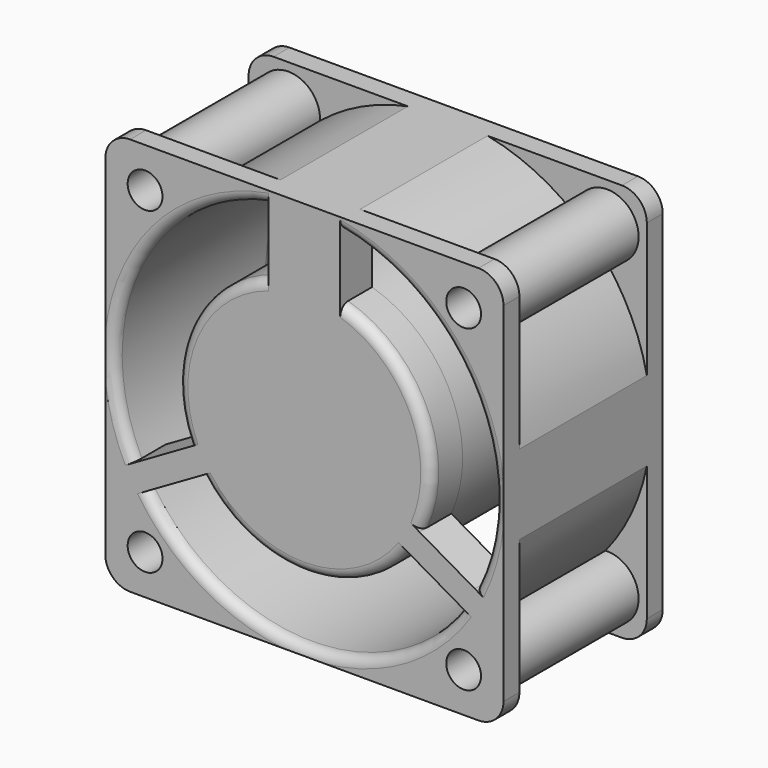
from build123d import *

# Parameters (mm, degrees)
F0_W         = 40
F0_H         = 40
F0_R         = 1.75
F0_R_2       = 19.1
F1_DEPTH     = 10
F3_DEPTH     = 8
F4_R         = 2.5
F6_DEPTH     = 4
F7_W         = 18
F7_H         = 12.7
F9_T6_ANGLE  = 120.5658801398
F9_T11_ANGLE = 120.5658801398
F9_T17_ANGLE = 120.5658801398
F9_T23_ANGLE = 120.5658801398
F9_T28_ANGLE = 131.5003349081
F9_T33_ANGLE = 131.5003349081
F9_T39_ANGLE = 131.5003349081
F9_T44_ANGLE = 120.4657257073
F9_T50_ANGLE = 120.4657257073
F9_T55_ANGLE = 86.6375868427
F9_T60_ANGLE = 127.6538287978
F9_T65_ANGLE = 127.6538287978
F9_T71_ANGLE = 127.6538287978
F9_T78_ANGLE = 33.8224519286
F9_T83_ANGLE = 33.8224519286


# Not quite as in the source:
# - a fillet or chamfer that OpenCascade refuses, or shapes differently, is made with other operations: its cross-section is extruded or revolved along the edge and cut away or added


with BuildPart() as f1:
    # F0 (on Front) → F1 (new body, symmetric)
    with BuildSketch(Plane.XZ):
        Rectangle(F0_W, F0_H)
        with Locations((-16, -16)):
            Circle(F0_R, mode=Mode.SUBTRACT)
        with Locations((16, -16)):
            Circle(F0_R, mode=Mode.SUBTRACT)
        with Locations((-16, 16)):
            Circle(F0_R, mode=Mode.SUBTRACT)
        Circle(F0_R_2, mode=Mode.SUBTRACT)
        with Locations((16, 16)):
            Circle(F0_R, mode=Mode.SUBTRACT)
    extrude(amount=F1_DEPTH, both=True)

    # F2 (on Front) → F3 (cut, symmetric)
    with BuildSketch(Plane.XZ):
        with BuildLine():
            ThreePointArc((-15.8567471072, 12.8282333616), (-18.2450640303, 18.2450640303), (-12.8282333616, 15.8567471072))
            ThreePointArc((-12.8282333616, 15.8567471072), (-8.6653906808, 18.463775463), (-4, 20))
            Line((-4, 20), (-4, 20.3960780544))
            Line((-4, 20.3960780544), (-20.3960780544, 20.3960780544))
            Line((-20.3960780544, 20.3960780544), (-20.3960780544, 4))
            Line((-20.3960780544, 4), (-20, 4))
            ThreePointArc((-20, 4), (-18.463775463, 8.6653906808), (-15.8567471072, 12.8282333616))
        make_face()
        with BuildLine():
            Line((20.3960780544, 4), (20.3960780544, 20.3960780544))
            Line((20.3960780544, 20.3960780544), (4, 20.3960780544))
            Line((4, 20.3960780544), (4, 20))
            ThreePointArc((4, 20), (8.6653906808, 18.463775463), (12.8282333616, 15.8567471072))
            ThreePointArc((12.8282333616, 15.8567471072), (18.2450640303, 18.2450640303), (15.8567471072, 12.8282333616))
            ThreePointArc((15.8567471072, 12.8282333616), (18.463775463, 8.6653906808), (20, 4))
            Line((20, 4), (20.3960780544, 4))
        make_face()
        with BuildLine():
            Line((-20.3960780544, -4), (-20.3960780544, -20.3960780544))
            Line((-20.3960780544, -20.3960780544), (-4, -20.3960780544))
            Line((-4, -20.3960780544), (-4, -20))
            ThreePointArc((-4, -20), (-8.6653906808, -18.463775463), (-12.8282333616, -15.8567471072))
            ThreePointArc((-12.8282333616, -15.8567471072), (-18.2450640303, -18.2450640303), (-15.8567471072, -12.8282333616))
            ThreePointArc((-15.8567471072, -12.8282333616), (-18.463775463, -8.6653906808), (-20, -4))
            Line((-20, -4), (-20.3960780544, -4))
        make_face()
        with BuildLine():
            Line((4, -20.3960780544), (20.3960780544, -20.3960780544))
            Line((20.3960780544, -20.3960780544), (20.3960780544, -4))
            Line((20.3960780544, -4), (20, -4))
            ThreePointArc((20, -4), (18.463775463, -8.6653906808), (15.8567471072, -12.8282333616))
            ThreePointArc((15.8567471072, -12.8282333616), (18.2450640303, -18.2450640303), (12.8282333616, -15.8567471072))
            ThreePointArc((12.8282333616, -15.8567471072), (8.6653906808, -18.463775463), (4, -20))
            Line((4, -20), (4, -20.3960780544))
        make_face()
    extrude(amount=F3_DEPTH, both=True, mode=Mode.SUBTRACT)

    # F4
    f4_edges = [f1.edges().sort_by_distance(p)[0] for p in [
        (20, -9, 20),
        (20, 9, 20),
        (20, -9, -20),
        (20, 9, -20),
        (-20, -9, 20),
        (-20, 9, 20),
        (-20, 9, -20),
        (-20, -9, -20),
    ]]
    fillet(f4_edges, radius=F4_R)

    # F5 (on face) → F6 (join)
    with BuildSketch(Plane.XZ.offset(10)):
        with BuildLine():
            Line((-3.6, 18.7576650999), (-3.6, 12.1790804251))
            ThreePointArc((-3.6, 12.1790804251), (-11.5533772944, 5.2734687913), (-11.5597385217, -5.2595099877))
            Line((-11.5597385217, -5.2595099877), (-17.1195297525, -8.4694569515))
            ThreePointArc((-17.1195297525, -8.4694569515), (-16.5410852123, -9.55), (-15.8945297525, -10.5912191908))
            Line((-15.8945297525, -10.5912191908), (-10.3347385217, -7.381272227))
            ThreePointArc((-10.3347385217, -7.381272227), (0, -12.7), (10.3347385217, -7.381272227))
            Line((10.3347385217, -7.381272227), (15.8945297525, -10.5912191908))
            ThreePointArc((15.8945297525, -10.5912191908), (16.5410852123, -9.55), (17.1195297525, -8.4694569515))
            Line((17.1195297525, -8.4694569515), (11.5597385217, -5.2595099877))
            ThreePointArc((11.5597385217, -5.2595099877), (11.5533772944, 5.2734687913), (3.6, 12.1790804251))
            Line((3.6, 12.1790804251), (3.6, 18.7576650999))
            ThreePointArc((3.6, 18.7576650999), (0, 19.1), (-3.6, 18.7576650999))
        make_face()
    extrude(amount=-F6_DEPTH)

    # F7 (on Right) → F8 (revolve)
    with BuildSketch(Plane.YZ):
        with Locations((1, 6.35)):
            Rectangle(F7_W, F7_H)
    revolve(axis=Axis((0, 1.2222109362, 0), (0, 1, 0)))

    # F9: fillet of radius 1 on 9 edges, made by hand

    # F9_s1 → F9_t2 (revolve, cut)
    with BuildSketch(Plane.YZ):
        with BuildLine():
            ThreePointArc((9, 12.7), (9.7071067812, 12.4071067812), (10, 11.7))
            Line((10, 11.7), (10, 12.7))
            Line((10, 12.7), (9, 12.7))
        make_face()
    revolve(axis=Axis((0, 10, 0), (0, 1, 0)), mode=Mode.SUBTRACT)


with BuildPart() as f9_tool4:
    # F9_s5 → F9_t6 (revolve)
    with BuildSketch(Plane(origin=(0, 0, 0), x_dir=(0, 1, 0), z_dir=(-0.5842341064, 0, -0.8115851828))):
        with BuildLine():
            ThreePointArc((-10, 11.7), (-9.7071067812, 12.4071067812), (-9, 12.7))
            Line((-9, 12.7), (-10, 12.7))
            Line((-10, 12.7), (-10, 11.7))
        make_face()
    revolve(axis=Axis((0, -10, 0), (0, -1, 0)), revolution_arc=F9_T6_ANGLE)

    split(bisect_by=Plane(origin=(-0.6125, 0, -1.0608811196), x_dir=(0, 1, 0), z_dir=(-0.5, 0, -0.8660254038)), keep=Keep.TOP)


with BuildPart() as f1_1:
    add(f1.part)

    # F9_t3: cut F9_tool4
    add(f9_tool4.part, mode=Mode.SUBTRACT)


with BuildPart() as f9_tool9:
    # F9_s10 → F9_t11 (revolve)
    with BuildSketch(Plane(origin=(0, 0, 0), x_dir=(0, 1, 0), z_dir=(-0.5842341064, 0, -0.8115851828))):
        with BuildLine():
            ThreePointArc((-10, 11.7), (-9.7071067812, 12.4071067812), (-9, 12.7))
            Line((-9, 12.7), (-10, 12.7))
            Line((-10, 12.7), (-10, 11.7))
        make_face()
    revolve(axis=Axis((0, -10, 0), (0, -1, 0)), revolution_arc=F9_T11_ANGLE)

    split(bisect_by=Plane.YZ.offset(3.6), keep=Keep.TOP)

    split(bisect_by=Plane(origin=(0.6125, 0, 1.0608811196), x_dir=(0, 1, 0), z_dir=(0.5, 0, 0.8660254038)), keep=Keep.TOP)


with BuildPart() as f1_2:
    add(f1_1.part)

    # F9_t8: cut F9_tool9
    add(f9_tool9.part, mode=Mode.SUBTRACT)


with BuildPart() as f9_tool15:
    # F9_s16 → F9_t17 (revolve)
    with BuildSketch(Plane(origin=(0, 0, 0), x_dir=(0, 1, 0), z_dir=(0.9959112122, 0, 0.0903374635))):
        with BuildLine():
            ThreePointArc((-10, 11.7), (-9.7071067812, 12.4071067812), (-9, 12.7))
            Line((-9, 12.7), (-10, 12.7))
            Line((-10, 12.7), (-10, 11.7))
        make_face()
    revolve(axis=Axis((0, -10, 0), (0, -1, 0)), revolution_arc=F9_T17_ANGLE)

    split(bisect_by=Plane(origin=(-0.6125, 0, 1.0608811196), x_dir=(0, 1, 0), z_dir=(-0.5, 0, 0.8660254038)), keep=Keep.TOP)

    split(bisect_by=Plane.YZ.offset(-3.6), keep=Keep.BOTTOM)


with BuildPart() as f1_3:
    add(f1_2.part)

    # F9_t14: cut F9_tool15
    add(f9_tool15.part, mode=Mode.SUBTRACT)


with BuildPart() as f9_tool21:
    # F9_s22 → F9_t23 (revolve)
    with BuildSketch(Plane(origin=(0, 0, 0), x_dir=(0, 1, 0), z_dir=(0.9959112122, 0, 0.0903374635))):
        with BuildLine():
            ThreePointArc((-10, 11.7), (-9.7071067812, 12.4071067812), (-9, 12.7))
            Line((-9, 12.7), (-10, 12.7))
            Line((-10, 12.7), (-10, 11.7))
        make_face()
    revolve(axis=Axis((0, -10, 0), (0, -1, 0)), revolution_arc=F9_T23_ANGLE)

    split(bisect_by=Plane(origin=(0.6125, 0, -1.0608811196), x_dir=(0, 1, 0), z_dir=(0.5, 0, -0.8660254038)), keep=Keep.TOP)


with BuildPart() as f1_4:
    add(f1_3.part)

    # F9_t20: cut F9_tool21
    add(f9_tool21.part, mode=Mode.SUBTRACT)


with BuildPart() as f9_tool26:
    # F9_s27 → F9_t28 (revolve)
    with BuildSketch(Plane(origin=(0, 0, 0), x_dir=(0, 1, 0), z_dir=(-0.4107161879, 0, 0.911763244))):
        with BuildLine():
            ThreePointArc((-10, 11.7), (-9.7071067812, 12.4071067812), (-9, 12.7))
            Line((-9, 12.7), (-10, 12.7))
            Line((-10, 12.7), (-10, 11.7))
        make_face()
    revolve(axis=Axis((0, -10, 0), (0, -1, 0)), revolution_arc=F9_T28_ANGLE)

    split(bisect_by=Plane(origin=(-0.6125, 0, 1.0608811196), x_dir=(0, 1, 0), z_dir=(-0.5, 0, 0.8660254038)), keep=Keep.TOP)


with BuildPart() as f1_5:
    add(f1_4.part)

    # F9_t25: cut F9_tool26
    add(f9_tool26.part, mode=Mode.SUBTRACT)


with BuildPart() as f9_tool31:
    # F9_s32 → F9_t33 (revolve)
    with BuildSketch(Plane(origin=(0, 0, 0), x_dir=(0, 1, 0), z_dir=(-0.4107161879, 0, 0.911763244))):
        with BuildLine():
            ThreePointArc((-10, 11.7), (-9.7071067812, 12.4071067812), (-9, 12.7))
            Line((-9, 12.7), (-10, 12.7))
            Line((-10, 12.7), (-10, 11.7))
        make_face()
    revolve(axis=Axis((0, -10, 0), (0, -1, 0)), revolution_arc=F9_T33_ANGLE)

    split(bisect_by=Plane(origin=(-0.6125, 0, -1.0608811196), x_dir=(0, 1, 0), z_dir=(-0.5, 0, -0.8660254038)), keep=Keep.TOP)

    split(bisect_by=Plane(origin=(0.6125, 0, -1.0608811196), x_dir=(0, 1, 0), z_dir=(0.5, 0, -0.8660254038)), keep=Keep.TOP)


with BuildPart() as f1_6:
    add(f1_5.part)

    # F9_t30: cut F9_tool31
    add(f9_tool31.part, mode=Mode.SUBTRACT)


with BuildPart() as f9_tool37:
    # F9_s38 → F9_t39 (revolve)
    with BuildSketch(Plane(origin=(0, 0, 0), x_dir=(0, 1, 0), z_dir=(-0.4107161879, 0, 0.911763244))):
        with BuildLine():
            ThreePointArc((-10, 11.7), (-9.7071067812, 12.4071067812), (-9, 12.7))
            Line((-9, 12.7), (-10, 12.7))
            Line((-10, 12.7), (-10, 11.7))
        make_face()
    revolve(axis=Axis((0, -10, 0), (0, -1, 0)), revolution_arc=F9_T39_ANGLE)

    split(bisect_by=Plane(origin=(0.6125, 0, 1.0608811196), x_dir=(0, 1, 0), z_dir=(0.5, 0, 0.8660254038)), keep=Keep.TOP)


with BuildPart() as f1_7:
    add(f1_6.part)

    # F9_t36: cut F9_tool37
    add(f9_tool37.part, mode=Mode.SUBTRACT)


with BuildPart() as f9_tool42:
    # F9_s43 → F9_t44 (revolve)
    with BuildSketch(Plane(origin=(0, 0, 0), x_dir=(0, 1, 0), z_dir=(0.998280369, 0, 0.0586200041))):
        with BuildLine():
            ThreePointArc((-10, 20.1), (-9.7071067812, 19.3928932188), (-9, 19.1))
            Line((-9, 19.1), (-10, 19.1))
            Line((-10, 19.1), (-10, 20.1))
        make_face()
    revolve(axis=Axis((0, -10, 0), (0, -1, 0)), revolution_arc=F9_T44_ANGLE)

    split(bisect_by=Plane(origin=(-0.6125, 0, 1.0608811196), x_dir=(0, 1, 0), z_dir=(-0.5, 0, 0.8660254038)), keep=Keep.TOP)

    split(bisect_by=Plane.YZ.offset(-3.6), keep=Keep.BOTTOM)


with BuildPart() as f1_8:
    add(f1_7.part)

    # F9_t41: cut F9_tool42
    add(f9_tool42.part, mode=Mode.SUBTRACT)


with BuildPart() as f9_tool48:
    # F9_s49 → F9_t50 (revolve)
    with BuildSketch(Plane(origin=(0, 0, 0), x_dir=(0, 1, 0), z_dir=(0.998280369, 0, 0.0586200041))):
        with BuildLine():
            ThreePointArc((-10, 20.1), (-9.7071067812, 19.3928932188), (-9, 19.1))
            Line((-9, 19.1), (-10, 19.1))
            Line((-10, 19.1), (-10, 20.1))
        make_face()
    revolve(axis=Axis((0, -10, 0), (0, -1, 0)), revolution_arc=F9_T50_ANGLE)

    split(bisect_by=Plane(origin=(0.6125, 0, -1.0608811196), x_dir=(0, 1, 0), z_dir=(0.5, 0, -0.8660254038)), keep=Keep.TOP)


with BuildPart() as f1_9:
    add(f1_8.part)

    # F9_t47: cut F9_tool48
    add(f9_tool48.part, mode=Mode.SUBTRACT)


with BuildPart() as f9_tool53:
    # F9_s54 → F9_t55 (revolve)
    with BuildSketch(Plane.XY):
        with BuildLine():
            ThreePointArc((20.1, -10), (19.3928932188, -9.7071067812), (19.1, -9))
            Line((19.1, -9), (19.1, -10))
            Line((19.1, -10), (20.1, -10))
        make_face()
    revolve(axis=Axis((0, -10, 0), (0, -1, 0)), revolution_arc=F9_T55_ANGLE)

    split(bisect_by=Plane.YZ.offset(3.6), keep=Keep.TOP)


with BuildPart() as f1_10:
    add(f1_9.part)

    # F9_t52: cut F9_tool53
    add(f9_tool53.part, mode=Mode.SUBTRACT)


with BuildPart() as f9_tool58:
    # F9_s59 → F9_t60 (revolve)
    with BuildSketch(Plane(origin=(0, 0, 0), x_dir=(0, 1, 0), z_dir=(-0.4410843216, 0, 0.8974656658))):
        with BuildLine():
            ThreePointArc((-10, 20.1), (-9.7071067812, 19.3928932188), (-9, 19.1))
            Line((-9, 19.1), (-10, 19.1))
            Line((-10, 19.1), (-10, 20.1))
        make_face()
    revolve(axis=Axis((0, -10, 0), (0, -1, 0)), revolution_arc=F9_T60_ANGLE)

    split(bisect_by=Plane(origin=(-0.6125, 0, 1.0608811196), x_dir=(0, 1, 0), z_dir=(-0.5, 0, 0.8660254038)), keep=Keep.TOP)


with BuildPart() as f1_11:
    add(f1_10.part)

    # F9_t57: cut F9_tool58
    add(f9_tool58.part, mode=Mode.SUBTRACT)


with BuildPart() as f9_tool63:
    # F9_s64 → F9_t65 (revolve)
    with BuildSketch(Plane(origin=(0, 0, 0), x_dir=(0, 1, 0), z_dir=(-0.4410843216, 0, 0.8974656658))):
        with BuildLine():
            ThreePointArc((-10, 20.1), (-9.7071067812, 19.3928932188), (-9, 19.1))
            Line((-9, 19.1), (-10, 19.1))
            Line((-10, 19.1), (-10, 20.1))
        make_face()
    revolve(axis=Axis((0, -10, 0), (0, -1, 0)), revolution_arc=F9_T65_ANGLE)

    split(bisect_by=Plane(origin=(-0.6125, 0, -1.0608811196), x_dir=(0, 1, 0), z_dir=(-0.5, 0, -0.8660254038)), keep=Keep.TOP)

    split(bisect_by=Plane(origin=(0.6125, 0, -1.0608811196), x_dir=(0, 1, 0), z_dir=(0.5, 0, -0.8660254038)), keep=Keep.TOP)


with BuildPart() as f1_12:
    add(f1_11.part)

    # F9_t62: cut F9_tool63
    add(f9_tool63.part, mode=Mode.SUBTRACT)


with BuildPart() as f9_tool69:
    # F9_s70 → F9_t71 (revolve)
    with BuildSketch(Plane(origin=(0, 0, 0), x_dir=(0, 1, 0), z_dir=(-0.4410843216, 0, 0.8974656658))):
        with BuildLine():
            ThreePointArc((-10, 20.1), (-9.7071067812, 19.3928932188), (-9, 19.1))
            Line((-9, 19.1), (-10, 19.1))
            Line((-10, 19.1), (-10, 20.1))
        make_face()
    revolve(axis=Axis((0, -10, 0), (0, -1, 0)), revolution_arc=F9_T71_ANGLE)

    split(bisect_by=Plane(origin=(0.6125, 0, 1.0608811196), x_dir=(0, 1, 0), z_dir=(0.5, 0, 0.8660254038)), keep=Keep.TOP)


with BuildPart() as f1_13:
    add(f1_12.part)

    # F9_t68: cut F9_tool69
    add(f9_tool69.part, mode=Mode.SUBTRACT)

    # F9_s73 → F9_t74 (revolve, cut)
    with BuildSketch(Plane.XY):
        with BuildLine():
            ThreePointArc((19.1, 9), (19.3928932188, 9.7071067812), (20.1, 10))
            Line((20.1, 10), (19.1, 10))
            Line((19.1, 10), (19.1, 9))
        make_face()
    revolve(axis=Axis((0, 10, 0), (0, -1, 0)), mode=Mode.SUBTRACT)


with BuildPart() as f9_tool76:
    # F9_s77 → F9_t78 (revolve)
    with BuildSketch(Plane(origin=(0, 0, 0), x_dir=(0, 1, 0), z_dir=(-0.5566212024, 0, -0.8307664154))):
        with BuildLine():
            ThreePointArc((-10, 20.1), (-9.7071067812, 19.3928932188), (-9, 19.1))
            Line((-9, 19.1), (-10, 19.1))
            Line((-10, 19.1), (-10, 20.1))
        make_face()
    revolve(axis=Axis((0, -10, 0), (0, -1, 0)), revolution_arc=F9_T78_ANGLE)

    split(bisect_by=Plane(origin=(-0.6125, 0, -1.0608811196), x_dir=(0, 1, 0), z_dir=(-0.5, 0, -0.8660254038)), keep=Keep.TOP)


with BuildPart() as f1_14:
    add(f1_13.part)

    # F9_t75: cut F9_tool76
    add(f9_tool76.part, mode=Mode.SUBTRACT)


with BuildPart() as f9_tool81:
    # F9_s82 → F9_t83 (revolve)
    with BuildSketch(Plane(origin=(0, 0, 0), x_dir=(0, 1, 0), z_dir=(-0.5566212024, 0, -0.8307664154))):
        with BuildLine():
            ThreePointArc((-10, 20.1), (-9.7071067812, 19.3928932188), (-9, 19.1))
            Line((-9, 19.1), (-10, 19.1))
            Line((-10, 19.1), (-10, 20.1))
        make_face()
    revolve(axis=Axis((0, -10, 0), (0, -1, 0)), revolution_arc=F9_T83_ANGLE)

    split(bisect_by=Plane(origin=(0.6125, 0, 1.0608811196), x_dir=(0, 1, 0), z_dir=(0.5, 0, 0.8660254038)), keep=Keep.TOP)


with BuildPart() as f1_15:
    add(f1_14.part)

    # F9_t80: cut F9_tool81
    add(f9_tool81.part, mode=Mode.SUBTRACT)


solid = f1_15.part
